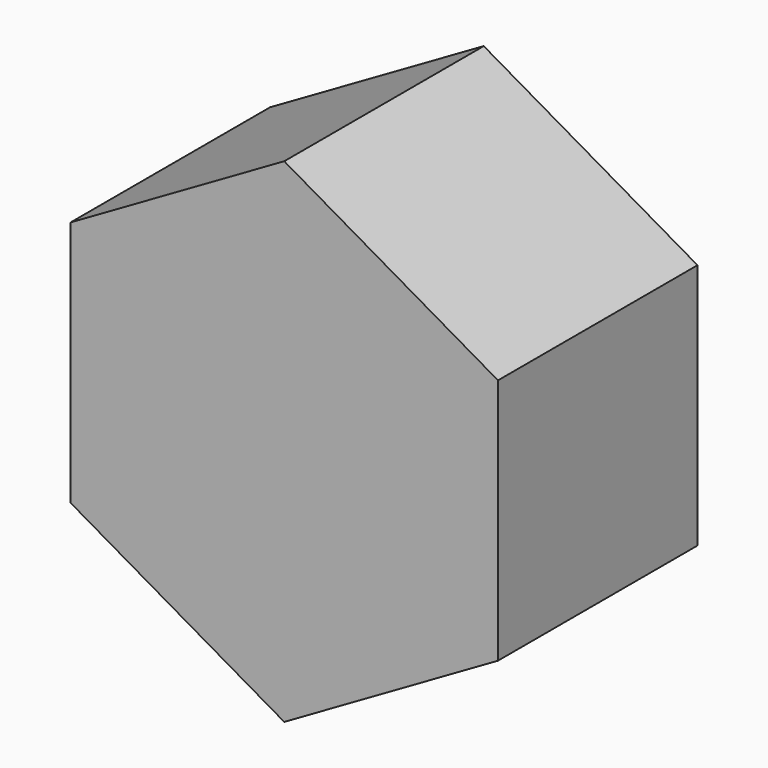
from build123d import *

# Parameters (mm, degrees)
F1_DEPTH = 8.334375


# Not quite as in the source:
# - a length typed as a fraction of an inch, garbled in the dataset ("3 / 203.2 mm" for 3/8 in), is restored


with BuildPart() as f1:
    # F0 (on Front) → F1 (new body)
    with BuildSketch(Plane.XZ):
        Polygon((7.14375, -4.1244459855), (7.14375, 4.1244459855), (0, 8.248891971), (-7.14375, 4.1244459855), (-7.14375, -4.1244459855), (0, -8.248891971), align=None)
    extrude(amount=F1_DEPTH)


solid = f1.part
